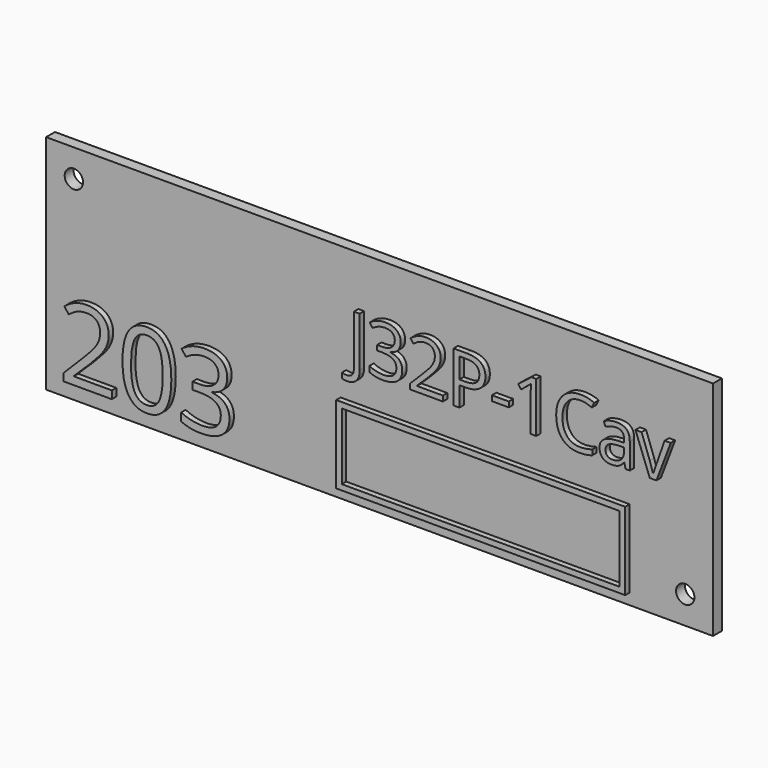
from build123d import *

# Parameters (mm, degrees)
F0_W         = 120
F0_H         = 40
F1_DEPTH     = 2
F3_D         = 3.3
F4_TEXT_SIZE = 12.6665787043
F5_DEPTH     = 1
F6_TEXT_SIZE = 18.5894526641
F7_DEPTH     = 1
F8_W         = 52
F8_H         = 14
F8_W_2       = 49.99999962
F8_H_2       = 11.99999962
F9_DEPTH     = 1


# Not quite as in the source:
# - Text() gives the source's letters only with a copy of the font that has no kerning and outlines rounded to 1/6400 em; it was checked with that copy


with BuildPart() as f1:
    # F0 (on Front) → F1 (new body)
    with BuildSketch(Plane.XZ):
        Rectangle(F0_W, F0_H)
    extrude(amount=F1_DEPTH)

    # F3 (through all)
    with Locations(Plane.XZ.offset(2)):
        with Locations((-55, 15), (55, -15)):
            Hole(F3_D / 2)

    # F4 (on face) → F5 (join)
    with BuildSketch(Plane.XZ.offset(2)):
        with Locations((-5, 2)):
            Text('J32P-1Cav', F4_TEXT_SIZE, font='Open Sans', text_align=(TextAlign.LEFT, TextAlign.BOTTOM))
    extrude(amount=F5_DEPTH)

    # F6 (on face) → F7 (join)
    with BuildSketch(Plane.XZ.offset(2)):
        with Locations((-57, -17)):
            Text('203', F6_TEXT_SIZE, font='Open Sans', text_align=(TextAlign.LEFT, TextAlign.BOTTOM))
    extrude(amount=F7_DEPTH)

    # F8 (on face) → F9 (join)
    with BuildSketch(Plane.XZ.offset(2)):
        with Locations((19, -11)):
            Rectangle(F8_W, F8_H)
        with Locations((19, -11)):
            Rectangle(F8_W_2, F8_H_2, mode=Mode.SUBTRACT)
    extrude(amount=F9_DEPTH)


solid = f1.part
